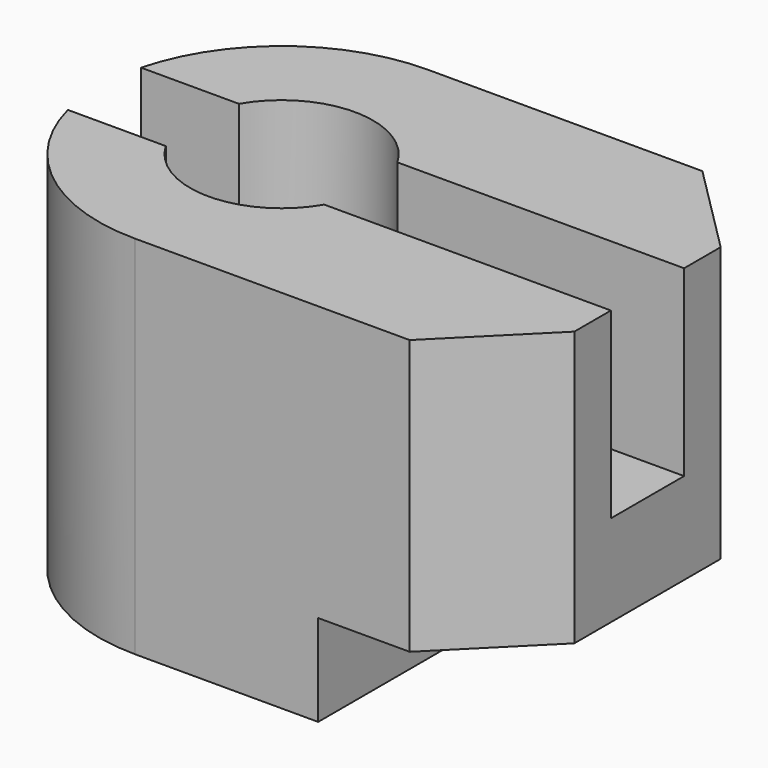
from build123d import *

# Parameters (mm, degrees)
F0_R     = 5
F1_DEPTH = 15
F3_DEPTH = 5
F4_DEPTH = 25
F6_DEPTH = 10


with BuildPart() as f1:
    # F0 (on Top) → F1 (new body)
    with BuildSketch(Plane.XY):
        with BuildLine():
            ThreePointArc((0, -10), (7.0710678119, -7.0710678119), (10, 0))
            ThreePointArc((10, 0), (7.0710678119, 7.0710678119), (0, 10))
            ThreePointArc((0, 10), (-10, 0), (0, -10))
        make_face()
        Circle(F0_R, mode=Mode.SUBTRACT)
        with BuildLine():
            ThreePointArc((0, 10), (7.0710678119, 7.0710678119), (10, 0))
            ThreePointArc((10, 0), (7.0710678119, -7.0710678119), (0, -10))
            Line((0, -10), (15, -10))
            Line((15, -10), (20, -5))
            Line((20, -5), (20, 5))
            Line((20, 5), (15, 10))
            Line((15, 10), (0, 10))
        make_face()
    extrude(amount=F1_DEPTH)

    # F2 (on face) → F3 (join)
    with BuildSketch(Plane(origin=(0, 0, 0), x_dir=(1, 0, 0), z_dir=(0, 0, -1))):
        with BuildLine():
            ThreePointArc((0, 10), (-10, 0), (0, -10))
            Line((0, -10), (10, -10))
            Line((10, -10), (10, 10))
            Line((10, 10), (0, 10))
        make_face()
    extrude(amount=F3_DEPTH)

    # F4 (cut): a face of the model
    f4_faces = [f1.faces().sort_by_distance(p)[0] for p in [
        (0, 0, 0),
    ]]
    extrude(f4_faces, amount=-F4_DEPTH, mode=Mode.SUBTRACT)

    # F5 (on face) → F6 (cut)
    with BuildSketch(Plane.XY.offset(15)):
        with BuildLine():
            ThreePointArc((-9.6824583655, 2.5), (-10, 0), (-9.6824583655, -2.5))
            Line((-9.6824583655, -2.5), (20, -2.5))
            Line((20, -2.5), (20, 2.5))
            Line((20, 2.5), (-9.6824583655, 2.5))
        make_face()
    extrude(amount=-F6_DEPTH, mode=Mode.SUBTRACT)


solid = f1.part
